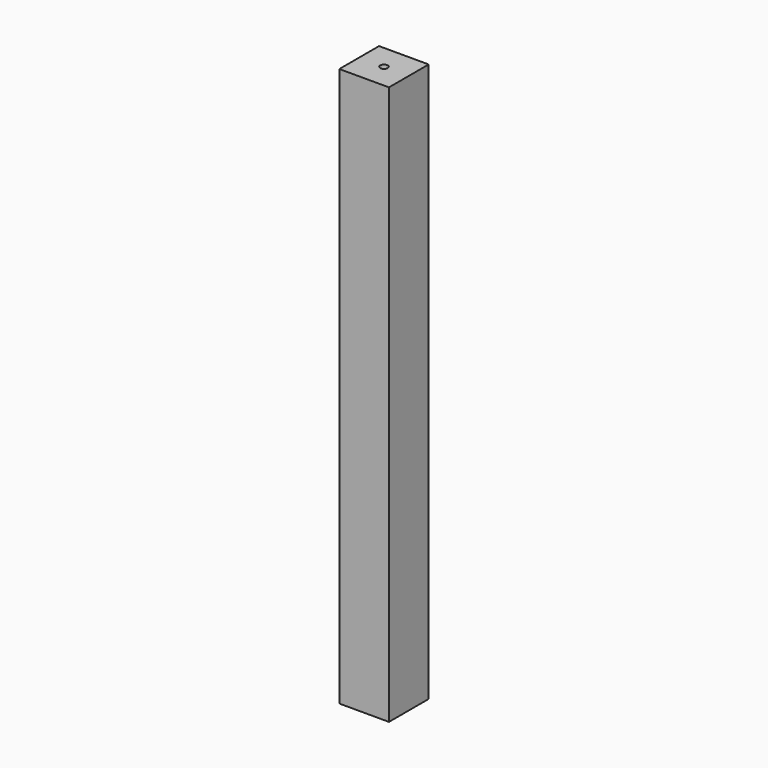
from build123d import *

# Parameters (mm, degrees)
F0_W     = 40
F0_H     = 40
F1_DEPTH = 450
F2_R     = 5
F3_DEPTH = 10
F4_DEPTH = 10
F5_R     = 3
F6_DEPTH = 12


# Not quite as in the source:
# - a feature of the source that left no trace in its solid (it failed there, or was rolled back) is left out


with BuildPart() as f1:
    # F0 (on Top) → F1 (new body)
    with BuildSketch(Plane.XY):
        with Locations((3.3165360987, -11.8447574973)):
            Rectangle(F0_W, F0_H)
    extrude(amount=F1_DEPTH)

    # F2 (on face) → F3 (join)
    with BuildSketch(Plane.XY.offset(450)):
        with Locations((3.3165360987, -11.8447574973)):
            Circle(F2_R)
    extrude(amount=F3_DEPTH)

    # F4 (cut): a face of the model
    f4_faces = [f1.faces().sort_by_distance(p)[0] for p in [
        (3.3165360987, -11.8447574973, 460),
    ]]
    extrude(f4_faces, amount=-F4_DEPTH, mode=Mode.SUBTRACT)

    # F5 (on face) → F6 (cut)
    with BuildSketch(Plane.XY.offset(450)):
        with Locations((3.3165360987, -11.8447574973)):
            Circle(F5_R)
    extrude(amount=-F6_DEPTH, mode=Mode.SUBTRACT)


solid = f1.part
